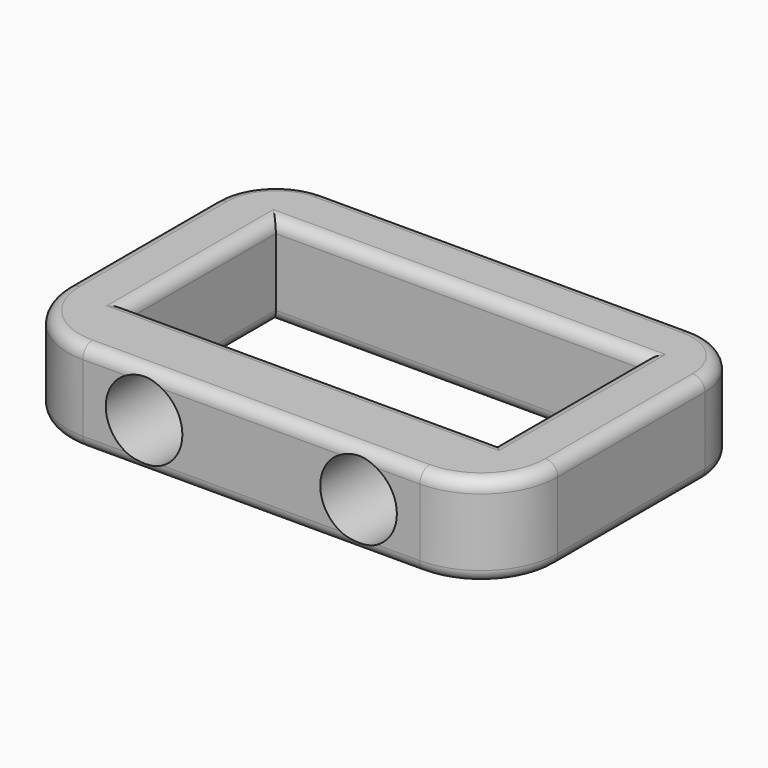
from build123d import *

# Parameters (mm, degrees)
F0_W           = 139.7
F0_H           = 38.1
F0_R           = 15.875
F1_DEPTH       = 15.875
F2_W           = 31.75
F2_H           = 38.1
F3_ANGLE       = 90
F4_W           = 25.4
F4_H           = 38.1
F5_DEPTH       = 76.2
F5_FACE_W      = 25.4
F5_FACE_H      = 38.1
F6_ANGLE       = 90
F7_W           = 25.4
F7_H           = 38.1
F8_DEPTH       = 76.2
F1_FACE1_W     = 31.75
F1_FACE1_H     = 38.1
F9_ANGLE       = 90
F10_W          = 25.4
F10_H          = 38.1
F11_DEPTH      = 76.2
F11_FACE_W     = 25.4
F11_FACE_H     = 38.1
F12_ANGLE      = 90
F13_DEPTH      = 76.2
F14_T1_DEPTH   = 152.4
F14_T3_DEPTH   = 76.2
F14_T5_DEPTH   = 139.7
F14_T8_ANGLE   = 90
F14_T10_ANGLE  = 90
F14_T12_ANGLE  = 90
F14_T14_ANGLE  = 90
F14_T16_ANGLE  = 90
F14_T18_ANGLE  = 90
F14_T20_ANGLE  = 90
F14_T22_ANGLE  = 90
F14_T27_DEPTH  = 165.1
F14_T31_DEPTH  = 88.9
F14_T38_DEPTH  = 165.1
F14_T42_DEPTH  = 88.9
F14_T49_DEPTH  = 165.1
F14_T53_DEPTH  = 88.9
F14_T60_DEPTH  = 165.1
F14_T64_DEPTH  = 88.9
F14_T71_DEPTH  = 88.9
F14_T75_DEPTH  = 165.1
F14_T82_DEPTH  = 88.9
F14_T86_DEPTH  = 165.1
F14_T93_DEPTH  = 165.1
F14_T97_DEPTH  = 88.9
F14_T104_DEPTH = 88.9
F14_T108_DEPTH = 165.1


# Not quite as in the source:
# - a fillet or chamfer that OpenCascade refuses, or shapes differently, is made with other operations: its cross-section is extruded or revolved along the edge and cut away or added


with BuildPart() as f1:
    # F0 (on Front) → F1 (new body, symmetric)
    with BuildSketch(Plane.XZ):
        Rectangle(F0_W, F0_H)
        with Locations((-44.45, 0)):
            Circle(F0_R, mode=Mode.SUBTRACT)
        with Locations((44.45, 0)):
            Circle(F0_R, mode=Mode.SUBTRACT)
    extrude(amount=F1_DEPTH, both=True)

    # F2 (on face) → F3 (revolve)
    with BuildSketch(Plane(origin=(-69.85, 0, 0), x_dir=(0, -1, 0), z_dir=(-1, 0, 0))):
        Rectangle(F2_W, F2_H)
    revolve(axis=Axis((-69.85, 15.875, 0), (0, 0, -1)), revolution_arc=F3_ANGLE)

    # F4 (on face) → F5 (join)
    with BuildSketch(Plane(origin=(0, 15.875, 0), x_dir=(-1, 0, 0), z_dir=(0, 1, 0))):
        with Locations((88.9, 0)):
            Rectangle(F4_W, F4_H)
    extrude(amount=F5_DEPTH)

    # F5_face (on face) → F6 (revolve)
    with BuildSketch(Plane(origin=(-88.9, 92.075, 0), x_dir=(-1, 0, 0), z_dir=(0, 1, 0))):
        Rectangle(F5_FACE_W, F5_FACE_H)
    revolve(axis=Axis((-76.2, 92.075, 0), (0, 0, -1)), revolution_arc=F6_ANGLE)

    # F7 (on face) → F8 (join, through all)
    with BuildSketch(Plane.YZ.offset(-76.2)):
        with Locations((104.775, 0)):
            Rectangle(F7_W, F7_H)
    extrude(amount=F8_DEPTH)

    # F1_face1 (on face) → F9 (revolve)
    with BuildSketch(Plane.YZ.offset(69.85)):
        Rectangle(F1_FACE1_W, F1_FACE1_H)
    revolve(axis=Axis((69.85, 15.875, 0), (0, 0, 1)), revolution_arc=F9_ANGLE)

    # F10 (on face) → F11 (join)
    with BuildSketch(Plane(origin=(0, 15.875, 0), x_dir=(-1, 0, 0), z_dir=(0, 1, 0))):
        with Locations((-88.9, 0)):
            Rectangle(F10_W, F10_H)
    extrude(amount=F11_DEPTH)

    # F11_face (on face) → F12 (revolve)
    with BuildSketch(Plane(origin=(88.9, 92.075, 0), x_dir=(-1, 0, 0), z_dir=(0, 1, 0))):
        Rectangle(F11_FACE_W, F11_FACE_H)
    revolve(axis=Axis((76.2, 92.075, 0), (0, 0, 1)), revolution_arc=F12_ANGLE)

    # F13 (add, through all): a face of the model
    f13_faces = [f1.faces().sort_by_distance(p)[0] for p in [
        (0, 104.775, 0),
    ]]
    extrude(f13_faces, amount=F13_DEPTH)

    # F14: fillet of radius 5.08 on 24 edges, made by hand

    # F14_s2 → F14_t1 (cut)
    with BuildSketch(Plane.YZ.offset(-76.2)):
        with BuildLine():
            ThreePointArc((10.795, 19.05), (14.3871024484, 17.5621024484), (15.875, 13.97))
            Line((15.875, 13.97), (15.875, 19.05))
            Line((15.875, 19.05), (10.795, 19.05))
        make_face()
        with BuildLine():
            ThreePointArc((92.075, 13.97), (93.5628975516, 17.5621024484), (97.155, 19.05))
            Line((97.155, 19.05), (92.075, 19.05))
            Line((92.075, 19.05), (92.075, 13.97))
        make_face()
        with BuildLine():
            ThreePointArc((112.395, 19.05), (115.9871024484, 17.5621024484), (117.475, 13.97))
            Line((117.475, 13.97), (117.475, 19.05))
            Line((117.475, 19.05), (112.395, 19.05))
        make_face()
        with BuildLine():
            ThreePointArc((112.395, -19.05), (115.9871024484, -17.5621024484), (117.475, -13.97))
            Line((117.475, -13.97), (117.475, -19.05))
            Line((117.475, -19.05), (112.395, -19.05))
        make_face()
        with BuildLine():
            ThreePointArc((10.795, -19.05), (14.3871024484, -17.5621024484), (15.875, -13.97))
            Line((15.875, -13.97), (15.875, -19.05))
            Line((15.875, -19.05), (10.795, -19.05))
        make_face()
        with BuildLine():
            ThreePointArc((97.155, -19.05), (93.5628975516, -17.5621024484), (92.075, -13.97))
            Line((92.075, -13.97), (92.075, -19.05))
            Line((92.075, -19.05), (97.155, -19.05))
        make_face()
    extrude(amount=F14_T1_DEPTH, mode=Mode.SUBTRACT)

    # F14_s4 → F14_t3 (cut)
    with BuildSketch(Plane.XZ.offset(-92.075)):
        with BuildLine():
            ThreePointArc((-81.28, 19.05), (-77.6878975516, 17.5621024484), (-76.2, 13.97))
            Line((-76.2, 13.97), (-76.2, 19.05))
            Line((-76.2, 19.05), (-81.28, 19.05))
        make_face()
        with BuildLine():
            ThreePointArc((81.28, 19.05), (77.6878975516, 17.5621024484), (76.2, 13.97))
            Line((76.2, 13.97), (76.2, 19.05))
            Line((76.2, 19.05), (81.28, 19.05))
        make_face()
        with BuildLine():
            ThreePointArc((-96.52, 19.05), (-100.1121024484, 17.5621024484), (-101.6, 13.97))
            Line((-101.6, 13.97), (-101.6, 19.05))
            Line((-101.6, 19.05), (-96.52, 19.05))
        make_face()
        with BuildLine():
            ThreePointArc((96.52, 19.05), (100.1121024484, 17.5621024484), (101.6, 13.97))
            Line((101.6, 13.97), (101.6, 19.05))
            Line((101.6, 19.05), (96.52, 19.05))
        make_face()
        with BuildLine():
            ThreePointArc((-96.52, -19.05), (-100.1121024484, -17.5621024484), (-101.6, -13.97))
            Line((-101.6, -13.97), (-101.6, -19.05))
            Line((-101.6, -19.05), (-96.52, -19.05))
        make_face()
        with BuildLine():
            ThreePointArc((96.52, -19.05), (100.1121024484, -17.5621024484), (101.6, -13.97))
            Line((101.6, -13.97), (101.6, -19.05))
            Line((101.6, -19.05), (96.52, -19.05))
        make_face()
        with BuildLine():
            ThreePointArc((-81.28, -19.05), (-77.6878975516, -17.5621024484), (-76.2, -13.97))
            Line((-76.2, -13.97), (-76.2, -19.05))
            Line((-76.2, -19.05), (-81.28, -19.05))
        make_face()
        with BuildLine():
            ThreePointArc((81.28, -19.05), (77.6878975516, -17.5621024484), (76.2, -13.97))
            Line((76.2, -13.97), (76.2, -19.05))
            Line((76.2, -19.05), (81.28, -19.05))
        make_face()
    extrude(amount=F14_T3_DEPTH, mode=Mode.SUBTRACT)

    # F14_s6 → F14_t5 (cut)
    with BuildSketch(Plane.YZ.offset(-69.85)):
        with BuildLine():
            ThreePointArc((-10.795, 19.05), (-14.3871024484, 17.5621024484), (-15.875, 13.97))
            Line((-15.875, 13.97), (-15.875, 19.05))
            Line((-15.875, 19.05), (-10.795, 19.05))
        make_face()
        with BuildLine():
            ThreePointArc((-10.795, -19.05), (-14.3871024484, -17.5621024484), (-15.875, -13.97))
            Line((-15.875, -13.97), (-15.875, -19.05))
            Line((-15.875, -19.05), (-10.795, -19.05))
        make_face()
    extrude(amount=F14_T5_DEPTH, mode=Mode.SUBTRACT)

    # F14_s7 → F14_t8 (revolve, cut)
    with BuildSketch(Plane.XZ.offset(-92.075)):
        with BuildLine():
            ThreePointArc((-96.52, 19.05), (-100.1121024484, 17.5621024484), (-101.6, 13.97))
            Line((-101.6, 13.97), (-101.6, 19.05))
            Line((-101.6, 19.05), (-96.52, 19.05))
        make_face()
    revolve(axis=Axis((-76.2, 92.075, 19.05), (0, 0, -1)), revolution_arc=F14_T8_ANGLE, mode=Mode.SUBTRACT)

    # F14_s9 → F14_t10 (revolve, cut)
    with BuildSketch(Plane.YZ.offset(-69.85)):
        with BuildLine():
            ThreePointArc((-10.795, 19.05), (-14.3871024484, 17.5621024484), (-15.875, 13.97))
            Line((-15.875, 13.97), (-15.875, 19.05))
            Line((-15.875, 19.05), (-10.795, 19.05))
        make_face()
    revolve(axis=Axis((-69.85, 15.875, 19.05), (0, 0, -1)), revolution_arc=F14_T10_ANGLE, mode=Mode.SUBTRACT)

    # F14_s11 → F14_t12 (revolve, cut)
    with BuildSketch(Plane.YZ.offset(69.85)):
        with BuildLine():
            ThreePointArc((-10.795, 19.05), (-14.3871024484, 17.5621024484), (-15.875, 13.97))
            Line((-15.875, 13.97), (-15.875, 19.05))
            Line((-15.875, 19.05), (-10.795, 19.05))
        make_face()
    revolve(axis=Axis((69.85, 15.875, 19.05), (0, 0, 1)), revolution_arc=F14_T12_ANGLE, mode=Mode.SUBTRACT)

    # F14_s13 → F14_t14 (revolve, cut)
    with BuildSketch(Plane.XZ.offset(-92.075)):
        with BuildLine():
            ThreePointArc((96.52, 19.05), (100.1121024484, 17.5621024484), (101.6, 13.97))
            Line((101.6, 13.97), (101.6, 19.05))
            Line((101.6, 19.05), (96.52, 19.05))
        make_face()
    revolve(axis=Axis((76.2, 92.075, 19.05), (0, 0, 1)), revolution_arc=F14_T14_ANGLE, mode=Mode.SUBTRACT)

    # F14_s15 → F14_t16 (revolve, cut)
    with BuildSketch(Plane.YZ.offset(-69.85)):
        with BuildLine():
            ThreePointArc((-10.795, -19.05), (-14.3871024484, -17.5621024484), (-15.875, -13.97))
            Line((-15.875, -13.97), (-15.875, -19.05))
            Line((-15.875, -19.05), (-10.795, -19.05))
        make_face()
    revolve(axis=Axis((-69.85, 15.875, -19.05), (0, 0, -1)), revolution_arc=F14_T16_ANGLE, mode=Mode.SUBTRACT)

    # F14_s17 → F14_t18 (revolve, cut)
    with BuildSketch(Plane.XZ.offset(-92.075)):
        with BuildLine():
            ThreePointArc((-96.52, -19.05), (-100.1121024484, -17.5621024484), (-101.6, -13.97))
            Line((-101.6, -13.97), (-101.6, -19.05))
            Line((-101.6, -19.05), (-96.52, -19.05))
        make_face()
    revolve(axis=Axis((-76.2, 92.075, -19.05), (0, 0, -1)), revolution_arc=F14_T18_ANGLE, mode=Mode.SUBTRACT)

    # F14_s19 → F14_t20 (revolve, cut)
    with BuildSketch(Plane.XZ.offset(-92.075)):
        with BuildLine():
            ThreePointArc((96.52, -19.05), (100.1121024484, -17.5621024484), (101.6, -13.97))
            Line((101.6, -13.97), (101.6, -19.05))
            Line((101.6, -19.05), (96.52, -19.05))
        make_face()
    revolve(axis=Axis((76.2, 92.075, -19.05), (0, 0, 1)), revolution_arc=F14_T20_ANGLE, mode=Mode.SUBTRACT)

    # F14_s21 → F14_t22 (revolve, cut)
    with BuildSketch(Plane.YZ.offset(69.85)):
        with BuildLine():
            ThreePointArc((-10.795, -19.05), (-14.3871024484, -17.5621024484), (-15.875, -13.97))
            Line((-15.875, -13.97), (-15.875, -19.05))
            Line((-15.875, -19.05), (-10.795, -19.05))
        make_face()
    revolve(axis=Axis((69.85, 15.875, -19.05), (0, 0, 1)), revolution_arc=F14_T22_ANGLE, mode=Mode.SUBTRACT)


with BuildPart() as f14_tool25:
    # F14_s26 → F14_t27 (new body)
    with BuildSketch(Plane.YZ.offset(-88.9)):
        with BuildLine():
            ThreePointArc((10.795, 19.05), (14.3871024484, 17.5621024484), (15.875, 13.97))
            Line((15.875, 13.97), (15.875, 19.05))
            Line((15.875, 19.05), (10.795, 19.05))
        make_face()
    extrude(amount=F14_T27_DEPTH)

    split(bisect_by=Plane.YZ.offset(-76.2), keep=Keep.BOTTOM)


with BuildPart() as f14_tool29:
    # F14_s30 → F14_t31 (new body)
    with BuildSketch(Plane.XZ.offset(-92.075)):
        with BuildLine():
            ThreePointArc((-81.28, 19.05), (-77.6878975516, 17.5621024484), (-76.2, 13.97))
            Line((-76.2, 13.97), (-76.2, 19.05))
            Line((-76.2, 19.05), (-81.28, 19.05))
        make_face()
    extrude(amount=F14_T31_DEPTH)

    split(bisect_by=Plane.XZ.offset(-15.875), keep=Keep.TOP)


with BuildPart() as f14_tool25_1:
    add(f14_tool25.part)

    # F14_t33: intersect F14_tool29
    add(f14_tool29.part, mode=Mode.INTERSECT)


with BuildPart() as f1_1:
    add(f1.part)

    # F14_t23: cut F14_tool25
    add(f14_tool25_1.part, mode=Mode.SUBTRACT)


with BuildPart() as f14_tool36:
    # F14_s37 → F14_t38 (new body)
    with BuildSketch(Plane.YZ.offset(-76.2)):
        with BuildLine():
            ThreePointArc((10.795, 19.05), (14.3871024484, 17.5621024484), (15.875, 13.97))
            Line((15.875, 13.97), (15.875, 19.05))
            Line((15.875, 19.05), (10.795, 19.05))
        make_face()
    extrude(amount=F14_T38_DEPTH)

    split(bisect_by=Plane.YZ.offset(76.2), keep=Keep.TOP)


with BuildPart() as f14_tool40:
    # F14_s41 → F14_t42 (new body)
    with BuildSketch(Plane.XZ.offset(-3.175)):
        with BuildLine():
            ThreePointArc((81.28, 19.05), (77.6878975516, 17.5621024484), (76.2, 13.97))
            Line((76.2, 13.97), (76.2, 19.05))
            Line((76.2, 19.05), (81.28, 19.05))
        make_face()
    extrude(amount=-F14_T42_DEPTH)

    split(bisect_by=Plane.XZ.offset(-15.875), keep=Keep.TOP)


with BuildPart() as f14_tool36_1:
    add(f14_tool36.part)

    # F14_t44: intersect F14_tool40
    add(f14_tool40.part, mode=Mode.INTERSECT)


with BuildPart() as f1_2:
    add(f1_1.part)

    # F14_t34: cut F14_tool36
    add(f14_tool36_1.part, mode=Mode.SUBTRACT)


with BuildPart() as f14_tool47:
    # F14_s48 → F14_t49 (new body)
    with BuildSketch(Plane.YZ.offset(76.2)):
        with BuildLine():
            ThreePointArc((92.075, 13.97), (93.5628975516, 17.5621024484), (97.155, 19.05))
            Line((97.155, 19.05), (92.075, 19.05))
            Line((92.075, 19.05), (92.075, 13.97))
        make_face()
    extrude(amount=-F14_T49_DEPTH)

    split(bisect_by=Plane.YZ.offset(-76.2), keep=Keep.BOTTOM)


with BuildPart() as f14_tool51:
    # F14_s52 → F14_t53 (new body)
    with BuildSketch(Plane.XZ.offset(-104.775)):
        with BuildLine():
            ThreePointArc((-81.28, 19.05), (-77.6878975516, 17.5621024484), (-76.2, 13.97))
            Line((-76.2, 13.97), (-76.2, 19.05))
            Line((-76.2, 19.05), (-81.28, 19.05))
        make_face()
    extrude(amount=F14_T53_DEPTH)

    split(bisect_by=Plane.XZ.offset(-92.075), keep=Keep.BOTTOM)


with BuildPart() as f14_tool47_1:
    add(f14_tool47.part)

    # F14_t55: intersect F14_tool51
    add(f14_tool51.part, mode=Mode.INTERSECT)


with BuildPart() as f1_3:
    add(f1_2.part)

    # F14_t45: cut F14_tool47
    add(f14_tool47_1.part, mode=Mode.SUBTRACT)


with BuildPart() as f14_tool58:
    # F14_s59 → F14_t60 (new body)
    with BuildSketch(Plane.YZ.offset(88.9)):
        with BuildLine():
            ThreePointArc((92.075, 13.97), (93.5628975516, 17.5621024484), (97.155, 19.05))
            Line((97.155, 19.05), (92.075, 19.05))
            Line((92.075, 19.05), (92.075, 13.97))
        make_face()
    extrude(amount=-F14_T60_DEPTH)

    split(bisect_by=Plane.YZ.offset(76.2), keep=Keep.TOP)


with BuildPart() as f14_tool62:
    # F14_s63 → F14_t64 (new body)
    with BuildSketch(Plane.XZ.offset(-15.875)):
        with BuildLine():
            ThreePointArc((81.28, 19.05), (77.6878975516, 17.5621024484), (76.2, 13.97))
            Line((76.2, 13.97), (76.2, 19.05))
            Line((76.2, 19.05), (81.28, 19.05))
        make_face()
    extrude(amount=-F14_T64_DEPTH)

    split(bisect_by=Plane.XZ.offset(-92.075), keep=Keep.BOTTOM)


with BuildPart() as f14_tool58_1:
    add(f14_tool58.part)

    # F14_t66: intersect F14_tool62
    add(f14_tool62.part, mode=Mode.INTERSECT)


with BuildPart() as f1_4:
    add(f1_3.part)

    # F14_t56: cut F14_tool58
    add(f14_tool58_1.part, mode=Mode.SUBTRACT)


with BuildPart() as f14_tool69:
    # F14_s70 → F14_t71 (new body)
    with BuildSketch(Plane.XZ.offset(-104.775)):
        with BuildLine():
            ThreePointArc((-81.28, -19.05), (-77.6878975516, -17.5621024484), (-76.2, -13.97))
            Line((-76.2, -13.97), (-76.2, -19.05))
            Line((-76.2, -19.05), (-81.28, -19.05))
        make_face()
    extrude(amount=F14_T71_DEPTH)

    split(bisect_by=Plane.XZ.offset(-92.075), keep=Keep.BOTTOM)


with BuildPart() as f14_tool73:
    # F14_s74 → F14_t75 (new body)
    with BuildSketch(Plane.YZ.offset(76.2)):
        with BuildLine():
            ThreePointArc((97.155, -19.05), (93.5628975516, -17.5621024484), (92.075, -13.97))
            Line((92.075, -13.97), (92.075, -19.05))
            Line((92.075, -19.05), (97.155, -19.05))
        make_face()
    extrude(amount=-F14_T75_DEPTH)

    split(bisect_by=Plane.YZ.offset(-76.2), keep=Keep.BOTTOM)


with BuildPart() as f14_tool69_1:
    add(f14_tool69.part)

    # F14_t77: intersect F14_tool73
    add(f14_tool73.part, mode=Mode.INTERSECT)


with BuildPart() as f1_5:
    add(f1_4.part)

    # F14_t67: cut F14_tool69
    add(f14_tool69_1.part, mode=Mode.SUBTRACT)


with BuildPart() as f14_tool80:
    # F14_s81 → F14_t82 (new body)
    with BuildSketch(Plane.XZ.offset(-92.075)):
        with BuildLine():
            ThreePointArc((-81.28, -19.05), (-77.6878975516, -17.5621024484), (-76.2, -13.97))
            Line((-76.2, -13.97), (-76.2, -19.05))
            Line((-76.2, -19.05), (-81.28, -19.05))
        make_face()
    extrude(amount=F14_T82_DEPTH)

    split(bisect_by=Plane.XZ.offset(-15.875), keep=Keep.TOP)


with BuildPart() as f14_tool84:
    # F14_s85 → F14_t86 (new body)
    with BuildSketch(Plane.YZ.offset(-88.9)):
        with BuildLine():
            ThreePointArc((10.795, -19.05), (14.3871024484, -17.5621024484), (15.875, -13.97))
            Line((15.875, -13.97), (15.875, -19.05))
            Line((15.875, -19.05), (10.795, -19.05))
        make_face()
    extrude(amount=F14_T86_DEPTH)

    split(bisect_by=Plane.YZ.offset(-76.2), keep=Keep.BOTTOM)


with BuildPart() as f14_tool80_1:
    add(f14_tool80.part)

    # F14_t88: intersect F14_tool84
    add(f14_tool84.part, mode=Mode.INTERSECT)


with BuildPart() as f1_6:
    add(f1_5.part)

    # F14_t78: cut F14_tool80
    add(f14_tool80_1.part, mode=Mode.SUBTRACT)


with BuildPart() as f14_tool91:
    # F14_s92 → F14_t93 (new body)
    with BuildSketch(Plane.YZ.offset(-76.2)):
        with BuildLine():
            ThreePointArc((10.795, -19.05), (14.3871024484, -17.5621024484), (15.875, -13.97))
            Line((15.875, -13.97), (15.875, -19.05))
            Line((15.875, -19.05), (10.795, -19.05))
        make_face()
    extrude(amount=F14_T93_DEPTH)

    split(bisect_by=Plane.YZ.offset(76.2), keep=Keep.TOP)


with BuildPart() as f14_tool95:
    # F14_s96 → F14_t97 (new body)
    with BuildSketch(Plane.XZ.offset(-3.175)):
        with BuildLine():
            ThreePointArc((81.28, -19.05), (77.6878975516, -17.5621024484), (76.2, -13.97))
            Line((76.2, -13.97), (76.2, -19.05))
            Line((76.2, -19.05), (81.28, -19.05))
        make_face()
    extrude(amount=-F14_T97_DEPTH)

    split(bisect_by=Plane.XZ.offset(-15.875), keep=Keep.TOP)


with BuildPart() as f14_tool91_1:
    add(f14_tool91.part)

    # F14_t99: intersect F14_tool95
    add(f14_tool95.part, mode=Mode.INTERSECT)


with BuildPart() as f1_7:
    add(f1_6.part)

    # F14_t89: cut F14_tool91
    add(f14_tool91_1.part, mode=Mode.SUBTRACT)


with BuildPart() as f14_tool102:
    # F14_s103 → F14_t104 (new body)
    with BuildSketch(Plane.XZ.offset(-15.875)):
        with BuildLine():
            ThreePointArc((81.28, -19.05), (77.6878975516, -17.5621024484), (76.2, -13.97))
            Line((76.2, -13.97), (76.2, -19.05))
            Line((76.2, -19.05), (81.28, -19.05))
        make_face()
    extrude(amount=-F14_T104_DEPTH)

    split(bisect_by=Plane.XZ.offset(-92.075), keep=Keep.BOTTOM)


with BuildPart() as f14_tool106:
    # F14_s107 → F14_t108 (new body)
    with BuildSketch(Plane.YZ.offset(88.9)):
        with BuildLine():
            ThreePointArc((97.155, -19.05), (93.5628975516, -17.5621024484), (92.075, -13.97))
            Line((92.075, -13.97), (92.075, -19.05))
            Line((92.075, -19.05), (97.155, -19.05))
        make_face()
    extrude(amount=-F14_T108_DEPTH)

    split(bisect_by=Plane.YZ.offset(76.2), keep=Keep.TOP)


with BuildPart() as f14_tool102_1:
    add(f14_tool102.part)

    # F14_t110: intersect F14_tool106
    add(f14_tool106.part, mode=Mode.INTERSECT)


with BuildPart() as f1_8:
    add(f1_7.part)

    # F14_t100: cut F14_tool102
    add(f14_tool102_1.part, mode=Mode.SUBTRACT)


solid = f1_8.part
